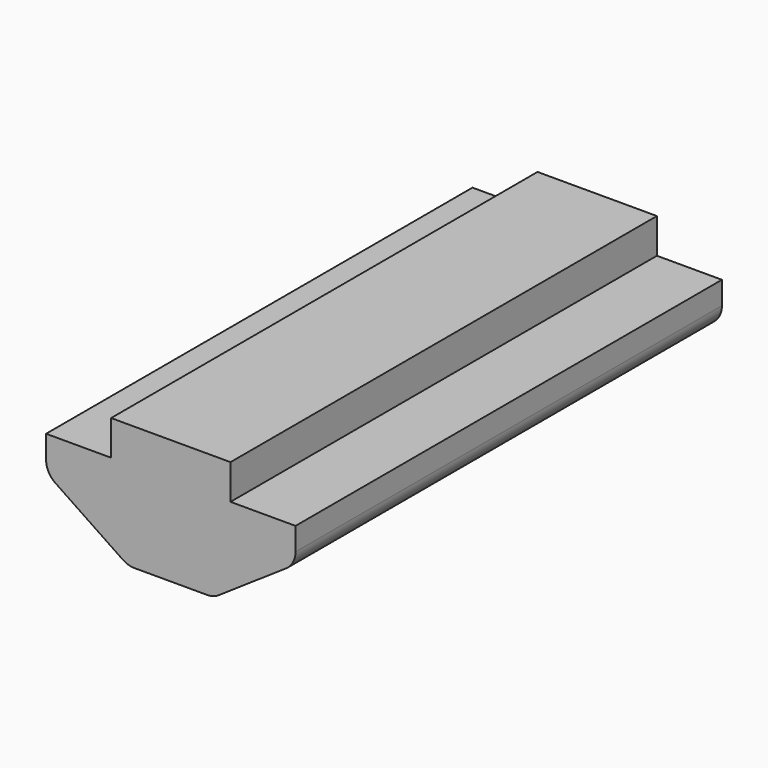
from build123d import *

# Parameters (mm, degrees)
F1_DEPTH = 31.75
F3_R     = 1.27


# Not quite as in the source:
# - a feature names something its author has since deleted; it is built from what else it names


with BuildPart() as f1:
    # F0 (on Front) → F1 (new body)
    with BuildSketch(Plane.XZ):
        Polygon((3.556, 2.0828), (-3.556, 2.0828), (-3.556, 0), (-7.4295, 0), (-7.4295, -2.032), (-2.54, -5.334), (2.54, -5.334), (7.4295, -2.032), (7.4295, 0), (3.556, 0), align=None)
    extrude(amount=F1_DEPTH)

    # F3
    f3_edges = [f1.edges().sort_by_distance(p)[0] for p in [
        (7.4295, -15.875, -2.032),
        (2.54, -15.875, -5.334),
        (-2.54, -15.875, -5.334),
        (-7.4295, -15.875, -2.032),
    ]]
    fillet(f3_edges, radius=F3_R)


solid = f1.part
